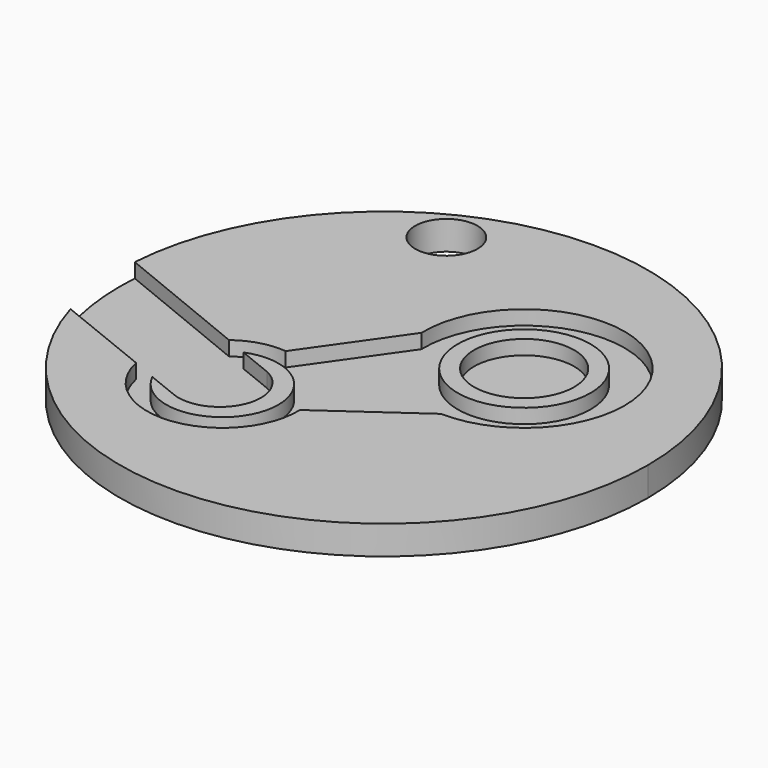
from build123d import *

# Parameters (mm, degrees)
F0_R     = 2.160588797
F1_DEPTH = 2
F0_R_2   = 4.5994043898
F2_DEPTH = 1
F0_R_3   = 3.4704819518
F3_DEPTH = 2


with BuildPart() as f1:
    # F0 (on Top) → F1 (new body)
    with BuildSketch(Plane.XY):
        with BuildLine():
            ThreePointArc((1.7638206969, 14.9172360687), (21.9354642074, 2.0549303863), (37.5805657932, 20.153684646))
            ThreePointArc((37.5805657932, 20.153684646), (19.9076326038, 38.4343937698), (1.0400371472, 21.3894316028))
            Line((1.0400371472, 21.3894316028), (10.7278591022, 17.4368359149))
            ThreePointArc((10.7278591022, 17.4368359149), (12.2433572681, 18.1926988563), (13.9304762706, 18.3399841189))
            Line((13.9304762706, 18.3399841189), (18.3288846165, 24.6035046875))
            ThreePointArc((18.3288846165, 24.6035046875), (30.1969763648, 29.7250639334), (25.0878613442, 17.8516097367))
            Line((25.0878613442, 17.8516097367), (18.846578896, 13.4367663413))
            ThreePointArc((18.846578896, 13.4367663413), (14.2233775819, 8.0711257596), (8.475728333, 12.2097991407))
            Line((8.475728333, 12.2097991407), (1.7638206969, 14.9172360687))
        make_face()
        with Locations((12.3943258077, 34.1789796948)):
            Circle(F0_R, mode=Mode.SUBTRACT)
    extrude(amount=F1_DEPTH)

    # F0 (on Top) → F2 (join)
    with BuildSketch(Plane.XY):
        with BuildLine():
            Line((10.7278591022, 17.4368359149), (1.0400371472, 21.3894316028))
            ThreePointArc((1.0400371472, 21.3894316028), (1.1115578041, 18.1208617268), (1.7638206969, 14.9172360687))
            Line((1.7638206969, 14.9172360687), (8.475728333, 12.2097991407))
            ThreePointArc((8.475728333, 12.2097991407), (14.2233775819, 8.0711257596), (18.846578896, 13.4367663413))
            Line((18.846578896, 13.4367663413), (25.0878613442, 17.8516097367))
            ThreePointArc((25.0878613442, 17.8516097367), (30.1969763648, 29.7250639334), (18.3288846165, 24.6035046875))
            Line((18.3288846165, 24.6035046875), (13.9304762706, 18.3399841189))
            ThreePointArc((13.9304762706, 18.3399841189), (12.2433572681, 18.1926988563), (10.7278591022, 17.4368359149))
        make_face()
        with BuildLine():
            ThreePointArc((12.2377891093, 16.798093915), (17.2918950944, 11.788760985), (10.1827690378, 11.476142332))
            Line((10.1827690378, 11.476142332), (12.3866147391, 10.587159116))
            ThreePointArc((12.3866147391, 10.587159116), (16.0771253181, 12.1102243495), (14.6324749478, 15.8321299564))
            Line((14.6324749478, 15.8321299564), (12.2377891093, 16.798093915))
        make_face(mode=Mode.SUBTRACT)
        with Locations((25.2813615695, 24.8042933578)):
            Circle(F0_R_2, mode=Mode.SUBTRACT)
    extrude(amount=F2_DEPTH)

    # F0 (on Top) → F3 (join)
    with BuildSketch(Plane.XY):
        with BuildLine():
            Line((12.3866147391, 10.587159116), (10.1827690378, 11.476142332))
            ThreePointArc((10.1827690378, 11.476142332), (17.2918950944, 11.788760985), (12.2377891093, 16.798093915))
            Line((12.2377891093, 16.798093915), (14.6324749478, 15.8321299564))
            ThreePointArc((14.6324749478, 15.8321299564), (16.0771253181, 12.1102243495), (12.3866147391, 10.587159116))
        make_face()
        with Locations((25.2813615695, 24.8042933578)):
            Circle(F0_R_2)
        with Locations((25.2813615695, 24.8042933578)):
            Circle(F0_R_3, mode=Mode.SUBTRACT)
    extrude(amount=F3_DEPTH)


with BuildPart() as f2:
    # F0 (on Top) → F2, piece 2 (new body)
    with BuildSketch(Plane.XY):
        with Locations((25.2813615695, 24.8042933578)):
            Circle(F0_R_3)
    extrude(amount=F2_DEPTH)


solid = Compound([f1.part, f2.part])
